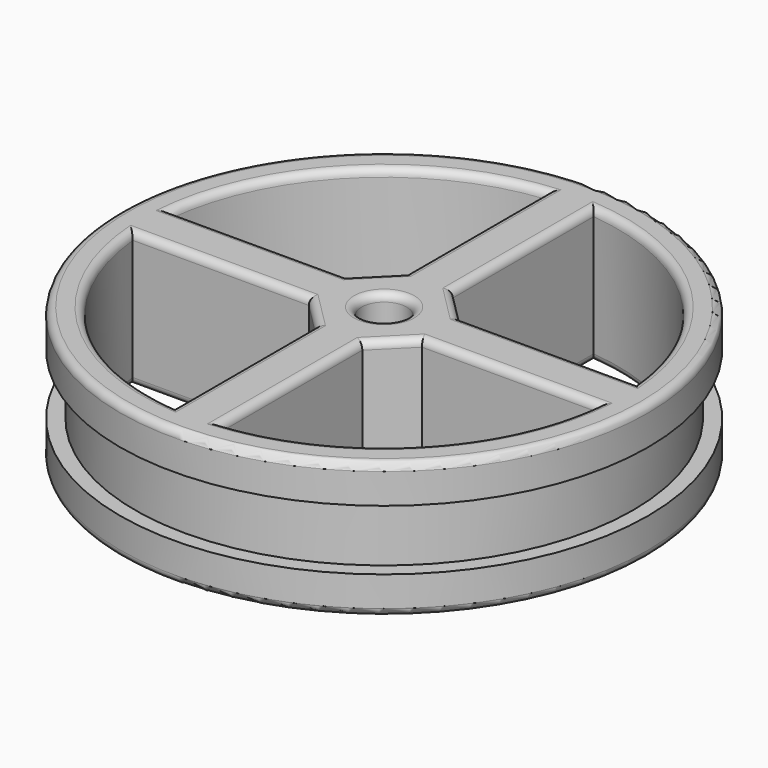
from build123d import *

# Parameters (mm, degrees)
F0_R     = 35
F0_R_2   = 3
F1_DEPTH = 18
F2_DEPTH = 10
F3_R     = 1
F5_D     = 3
F6_W     = 5.9583846331
F6_H     = 8
F6_W_2   = 2.0416153669


# Not quite as in the source:
# - a feature names something its author has since deleted; it is built from what else it names


with BuildPart() as f1:
    # F0 (on Top) → F1 (new body)
    with BuildSketch(Plane.XY):
        Circle(F0_R)
        with BuildLine():
            ThreePointArc((30.8439463391, 3.1066017178), (30.9609620047, 1.5552593818), (31, 0))
            ThreePointArc((31, 0), (30.9609620047, -1.5552593818), (30.8439463391, -3.1066017178))
            ThreePointArc((30.8439463391, -3.1066017178), (21.9203102168, -21.9203102168), (3.1066017178, -30.8439463391))
            ThreePointArc((3.1066017178, -30.8439463391), (0, -31), (-3.1066017178, -30.8439463391))
            ThreePointArc((-3.1066017178, -30.8439463391), (-21.9203102168, -21.9203102168), (-30.8439463391, -3.1066017178))
            ThreePointArc((-30.8439463391, -3.1066017178), (-31, 0), (-30.8439463391, 3.1066017178))
            ThreePointArc((-30.8439463391, 3.1066017178), (-21.9203102168, 21.9203102168), (-3.1066017178, 30.8439463391))
            ThreePointArc((-3.1066017178, 30.8439463391), (0, 31), (3.1066017178, 30.8439463391))
            ThreePointArc((3.1066017178, 30.8439463391), (21.9203102168, 21.9203102168), (30.8439463391, 3.1066017178))
        make_face(mode=Mode.SUBTRACT)
        with BuildLine():
            ThreePointArc((30.8439463391, -3.1066017178), (30.9609620047, -1.5552593818), (31, 0))
            ThreePointArc((31, 0), (30.9609620047, 1.5552593818), (30.8439463391, 3.1066017178))
            Line((30.8439463391, 3.1066017178), (7.5, 3.1066017178))
            Line((7.5, 3.1066017178), (7.5, -3.1066017178))
            Line((7.5, -3.1066017178), (30.8439463391, -3.1066017178))
        make_face()
        with BuildLine():
            Line((3.1066017178, 7.5), (3.1066017178, 30.8439463391))
            ThreePointArc((3.1066017178, 30.8439463391), (0, 31), (-3.1066017178, 30.8439463391))
            Line((-3.1066017178, 30.8439463391), (-3.1066017178, 7.5))
            Line((-3.1066017178, 7.5), (3.1066017178, 7.5))
        make_face()
        with BuildLine():
            Line((-7.5, 3.1066017178), (-30.8439463391, 3.1066017178))
            ThreePointArc((-30.8439463391, 3.1066017178), (-31, 0), (-30.8439463391, -3.1066017178))
            Line((-30.8439463391, -3.1066017178), (-7.5, -3.1066017178))
            Line((-7.5, -3.1066017178), (-7.5, 3.1066017178))
        make_face()
        with BuildLine():
            ThreePointArc((-3.1066017178, -30.8439463391), (0, -31), (3.1066017178, -30.8439463391))
            Line((3.1066017178, -30.8439463391), (3.1066017178, -7.5))
            Line((3.1066017178, -7.5), (-3.1066017178, -7.5))
            Line((-3.1066017178, -7.5), (-3.1066017178, -30.8439463391))
        make_face()
        Polygon((7.5, -3.1066017178), (7.5, 3.1066017178), (3.1066017178, 7.5), (-3.1066017178, 7.5), (-7.5, 3.1066017178), (-7.5, -3.1066017178), (-3.1066017178, -7.5), (3.1066017178, -7.5), align=None)
        Circle(F0_R_2, mode=Mode.SUBTRACT)
    extrude(amount=F1_DEPTH)

    # F0 (on Top) → F2 (join)
    with BuildSketch(Plane.XY):
        Polygon((7.5, -3.1066017178), (7.5, 3.1066017178), (3.1066017178, 7.5), (-3.1066017178, 7.5), (-7.5, 3.1066017178), (-7.5, -3.1066017178), (-3.1066017178, -7.5), (3.1066017178, -7.5), align=None)
        Circle(F0_R_2, mode=Mode.SUBTRACT)
    extrude(amount=-F2_DEPTH)

    # F3
    f3_edges = [f1.edges().sort_by_distance(p)[0] for p in [
        (-35, 0, 18),
        (21.92031, -21.92031, 18),
        (3.106602, -19.171973, 18),
        (5.303301, -5.303301, 18),
        (19.171973, -3.106602, 18),
        (-3.106602, -19.171973, 18),
        (-21.92031, -21.92031, 18),
        (-19.171973, -3.106602, 18),
        (-5.303301, -5.303301, 18),
        (-19.171973, 3.106602, 18),
        (-21.92031, 21.92031, 18),
        (-3.106602, 19.171973, 18),
        (-5.303301, 5.303301, 18),
        (3.106602, 19.171973, 18),
        (21.92031, 21.92031, 18),
        (19.171973, 3.106602, 18),
        (5.303301, 5.303301, 18),
        (-3, 0, 18),
        (0, -7.5, -10),
        (5.303301, -5.303301, -10),
        (7.5, 0, -10),
        (5.303301, 5.303301, -10),
        (0, 7.5, -10),
        (-5.303301, 5.303301, -10),
        (-7.5, 0, -10),
        (-5.303301, -5.303301, -10),
        (-35, 0, 0),
        (-3.106602, 19.171973, 0),
        (3.106602, 19.171973, 0),
        (19.171973, 3.106602, 0),
        (19.171973, -3.106602, 0),
        (3.106602, -19.171973, 0),
        (-3.106602, -19.171973, 0),
        (-19.171973, -3.106602, 0),
        (21.92031, 21.92031, 0),
        (21.92031, -21.92031, 0),
        (-21.92031, -21.92031, 0),
        (-21.92031, 21.92031, 0),
        (-19.171973, 3.106602, 0),
    ]]
    fillet(f3_edges, radius=F3_R)

    # F5 (through all)
    with Locations(Plane(origin=(0, 7.5, 0), x_dir=(-1, 0, 0), z_dir=(0, 1, 0))):
        with Locations((0, -3.75)):
            Hole(F5_D / 2)

    # F6 (on Front) → F7 (revolve, cut)
    with BuildSketch(Plane.XZ):
        with Locations((-38.0208076835, 9)):
            Rectangle(F6_W, F6_H)
        with Locations((-34.0208076835, 9)):
            Rectangle(F6_W_2, F6_H)
    revolve(axis=Axis((0, 0, 17), (0, 0, 1)), mode=Mode.SUBTRACT)


solid = f1.part
